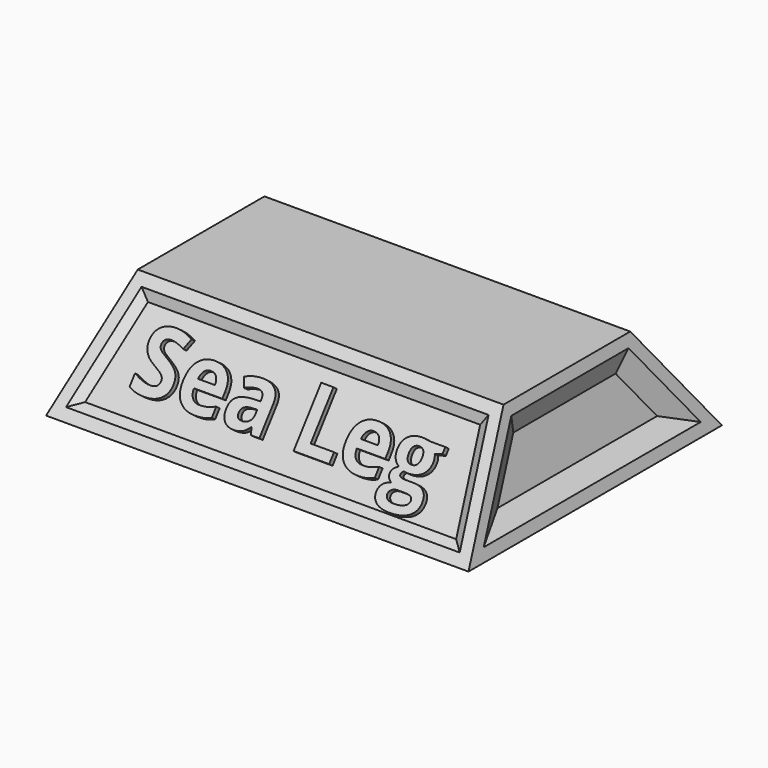
from build123d import *

# Parameters (mm, degrees)
F1_DEPTH      = 40
F3_DEPTH      = 30.001
F6_DEPTH      = 2
F6_TAPER      = 60
F9_DEPTH      = 1
F9_TAPER      = 60
F11_DEPTH     = 1
F11_TAPER     = 60
F12_TEXT_SIZE = 15.2777777778
F14_DEPTH     = 1
F13_TEXT_SIZE = 15.2777777778
F15_DEPTH     = 1


# Not quite as in the source:
# - Text() gives the source's letters only with a copy of the font that has no kerning and outlines rounded to 1/6400 em; it was checked with that copy


with BuildPart() as f1:
    # F0 (on Right) → F1 (new body)
    with BuildSketch(Plane.YZ):
        Polygon((0, 0), (0, 20), (-15, 20), (-30, 0), align=None)
    extrude(amount=-F1_DEPTH)

    # F2 (on Front) → F3 (cut, through all)
    with BuildSketch(Plane.XZ):
        Polygon((-40, 20), (-40, 0), (-34.6410161514, 20), align=None)
    extrude(amount=F3_DEPTH, mode=Mode.SUBTRACT)

    # F4: F1 across face


with BuildPart() as f1_1:
    add(f1.part)
    add(f1.part.mirror(Plane(origin=(-18.692317182, 0, 9.7606774343), x_dir=(-1, 0, 0), z_dir=(0, 1, 0))))

    # F5 (on face) → F6 (cut)
    with BuildSketch(Plane(origin=(-37.3205080757, 0, 10), x_dir=(0, -1, 0), z_dir=(-0.9659258263, 0, 0.2588190451))):
        Polygon((25.6895828532, -8.1527614966), (13.8771385255, 8.1527614966), (-13.8771385255, 8.1527614966), (-25.6895828532, -8.1527614966), align=None)
    extrude(amount=-F6_DEPTH, taper=F6_TAPER, mode=Mode.SUBTRACT)

    # F7: F1 across face


with BuildPart() as f1_2:
    add(f1_1.part)
    add(f1_1.part.mirror(Plane(origin=(0, 0, 8.8888888889), x_dir=(0, 1, 0), z_dir=(1, 0, 0))))

    # F8 (on face) → F9 (cut)
    with BuildSketch(Plane(origin=(0, -19.2, 14.4), x_dir=(1, 0, 0), z_dir=(0, -0.8, 0.6))):
        Polygon((37.2784321606, -15.8), (32.8626294693, 4.8), (-32.8626294693, 4.8), (-37.2784321606, -15.8), align=None)
    extrude(amount=-F9_DEPTH, taper=F9_TAPER, mode=Mode.SUBTRACT)

    # F10 (on face) → F11 (cut)
    with BuildSketch(Plane(origin=(0, 19.2, 14.4), x_dir=(-1, 0, 0), z_dir=(0, 0.8, 0.6))):
        Polygon((37.2784321606, -15.8), (32.8626294693, 4.8), (-32.8626294693, 4.8), (-37.2784321606, -15.8), align=None)
    extrude(amount=-F11_DEPTH, taper=F11_TAPER, mode=Mode.SUBTRACT)

    # F12 (on face) → F14 (join)
    with BuildSketch(Plane(origin=(0, -18.4, 13.8), x_dir=(1, 0, 0), z_dir=(0, -0.8, 0.6))):
        with Locations((-28.8702256944, -10.2129767342)):
            Text('Sea Leg', F12_TEXT_SIZE, font='Open Sans', font_style=FontStyle.BOLD, text_align=(TextAlign.LEFT, TextAlign.BOTTOM))
    extrude(amount=F14_DEPTH)

    # F13 (on face) → F15 (join)
    with BuildSketch(Plane(origin=(0, 18.4, 13.8), x_dir=(-1, 0, 0), z_dir=(0, 0.8, 0.6))):
        with Locations((-28.8702256944, -10.1767038154)):
            Text('Sea Leg', F13_TEXT_SIZE, font='Open Sans', font_style=FontStyle.BOLD, text_align=(TextAlign.LEFT, TextAlign.BOTTOM))
    extrude(amount=F15_DEPTH)


solid = f1_2.part
